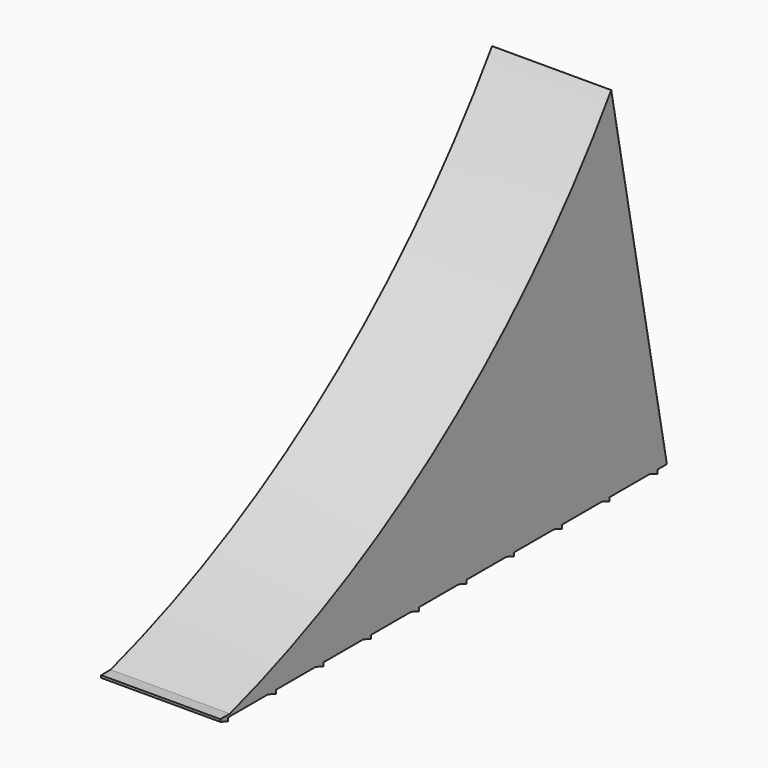
from build123d import *

# Parameters (mm, degrees)
F1_DEPTH = 25


with BuildPart() as f1:
    # F0 (on Right) → F1 (new body, symmetric)
    with BuildSketch(Plane.YZ):
        Polygon((-100, -75), (-100, -74), (-105, -74), (-105, -75), (-100.8787838708, -75), align=None)
        with BuildLine():
            Line((100, -75), (100, 75))
            ThreePointArc((100, 75), (12.7497178819, -16.6137152777), (-100, -74))
            Line((-100, -74), (-100, -75))
            Line((-100, -75), (-80, -75))
            Line((-80, -75), (-75.8787838708, -75))
            Line((-75.8787838708, -75), (-55, -75))
            Line((-55, -75), (-50.8787838708, -75))
            Line((-50.8787838708, -75), (-30, -75))
            Line((-30, -75), (-25.8787838708, -75))
            Line((-25.8787838708, -75), (-5, -75))
            Line((-5, -75), (-0.8787838708, -75))
            Line((-0.8787838708, -75), (20, -75))
            Line((20, -75), (24.1212161292, -75))
            Line((24.1212161292, -75), (45, -75))
            Line((45, -75), (49.1212161292, -75))
            Line((49.1212161292, -75), (70, -75))
            Line((70, -75), (74.1212161292, -75))
            Line((74.1212161292, -75), (95, -75))
            Line((95, -75), (99.1212161292, -75))
            Line((99.1212161292, -75), (100, -75))
        make_face()
        Polygon((129.1570463707, -75), (100, 75), (100, -75), (120, -75), (124.1212161292, -75), align=None)
        Polygon((-100.8787838708, -75), (-105, -75), (-100.8787838708, -76.5), align=None)
        Polygon((-75.8787838708, -75), (-80, -75), (-75.8787838708, -76.5), align=None)
        Polygon((-50.8787838708, -75), (-55, -75), (-50.8787838708, -76.5), align=None)
        Polygon((-25.8787838708, -75), (-30, -75), (-25.8787838708, -76.5), align=None)
        Polygon((-0.8787838708, -75), (-5, -75), (-0.8787838708, -76.5), align=None)
        Polygon((24.1212161292, -76.5), (24.1212161292, -75), (20, -75), align=None)
        Polygon((49.1212161292, -76.5), (49.1212161292, -75), (45, -75), align=None)
        Polygon((74.1212161292, -76.5), (74.1212161292, -75), (70, -75), align=None)
        Polygon((99.1212161292, -76.5), (99.1212161292, -75), (95, -75), align=None)
        Polygon((124.1212161292, -75), (120, -75), (124.1212161292, -76.5), align=None)
    extrude(amount=F1_DEPTH, both=True)


solid = f1.part
